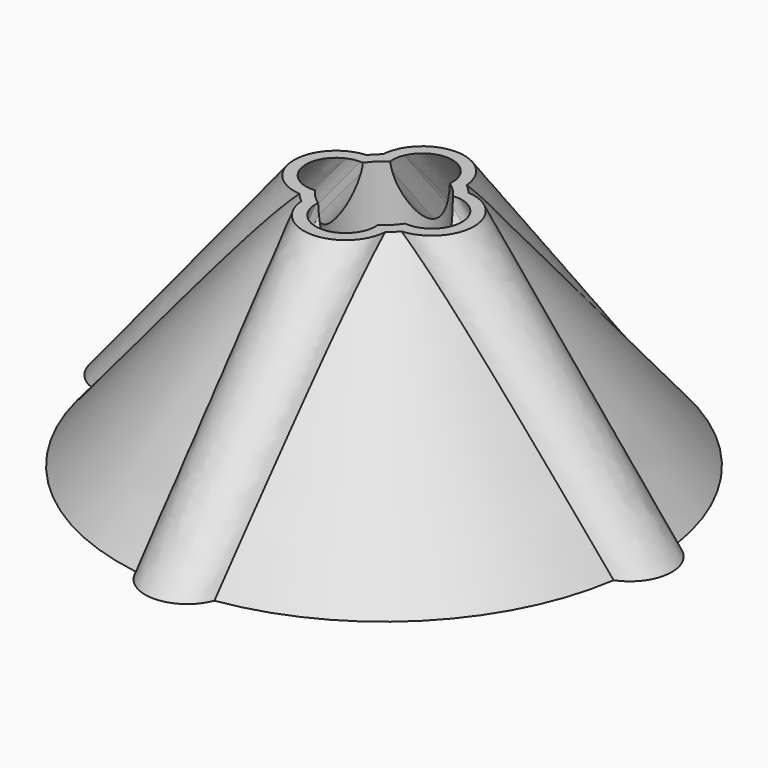
from build123d import *

# Parameters (mm, degrees)
F7_COUNT  = 4
F8_COUNT  = 4
F10_R     = 0.9
F11_DEPTH = 4


with BuildPart() as f1:
    # F0 (on Front) → F1 (revolve)
    with BuildSketch(Plane.XZ):
        Polygon((-0.8, 0), (-0.8, 4), (-1.1, 4), (-4.4, 0), align=None)
    revolve(axis=Axis((0, 0, 2), (0, 0, 1)))

    # F5: sweep along a path in F4
    with BuildLine(Plane(origin=(0, 0, 0), x_dir=(0, -1, 0), z_dir=(-1, 0, 0))) as f5_path:
        Line((-4.4, 0), (-1.1, 4))
    # F2 (on face) → F5 (sweep)
    with BuildSketch(Plane.XY.offset(4)):
        with BuildLine():
            ThreePointArc((0.4582575695, 1), (0.5830784403, 0.9327483757), (0.6982120022, 0.85))
            ThreePointArc((0.6982120022, 0.85), (0, 1.5), (-0.6982120022, 0.85))
            ThreePointArc((-0.6982120022, 0.85), (-0.5830784403, 0.9327483757), (-0.4582575695, 1))
            ThreePointArc((-0.4582575695, 1), (0, 1.3), (0.4582575695, 1))
        make_face()
        with BuildLine():
            ThreePointArc((-0.4582575695, 1), (-0.5830784403, 0.9327483757), (-0.6982120022, 0.85))
            ThreePointArc((-0.6982120022, 0.85), (-0.6873150882, 0.667342661), (-0.6294528874, 0.49375))
            ThreePointArc((-0.6294528874, 0.49375), (-0.5572758185, 0.5739718304), (-0.4749588798, 0.64375))
            ThreePointArc((-0.4749588798, 0.64375), (-0.49945145, 0.823414719), (-0.4582575695, 1))
        make_face()
        with BuildLine():
            ThreePointArc((-0.6294528874, 0.49375), (0, 0.1), (0.6294528874, 0.49375))
            ThreePointArc((0.6294528874, 0.49375), (0.5572758185, 0.5739718304), (0.4749588798, 0.64375))
            ThreePointArc((0.4749588798, 0.64375), (0, 0.3), (-0.4749588798, 0.64375))
            ThreePointArc((-0.4749588798, 0.64375), (-0.5572758185, 0.5739718304), (-0.6294528874, 0.49375))
        make_face()
        with BuildLine():
            ThreePointArc((0.6294528874, 0.49375), (0.6821352583, 0.6428647417), (0.7, 0.8))
            ThreePointArc((0.7, 0.8), (0.6995528577, 0.8250159796), (0.6982120022, 0.85))
            ThreePointArc((0.6982120022, 0.85), (0.5830784403, 0.9327483757), (0.4582575695, 1))
            ThreePointArc((0.4582575695, 1), (0.4894531565, 0.9021548218), (0.5, 0.8))
            ThreePointArc((0.5, 0.8), (0.4937000303, 0.7208780685), (0.4749588798, 0.64375))
            ThreePointArc((0.4749588798, 0.64375), (0.5572758185, 0.5739718304), (0.6294528874, 0.49375))
        make_face()
    sweep(path=f5_path.line)

    # F6: sweep along a path in F4
    with BuildLine(Plane(origin=(0, 0, 0), x_dir=(0, -1, 0), z_dir=(-1, 0, 0))) as f6_path:
        Line((-4.4, 0), (-1.1, 4))
    # F2 (on face) → F6 (sweep, cut)
    with BuildSketch(Plane.XY.offset(4)):
        with BuildLine():
            ThreePointArc((-0.4582575695, 1), (0, 1.1), (0.4582575695, 1))
            ThreePointArc((0.4582575695, 1), (0, 1.3), (-0.4582575695, 1))
        make_face()
        with BuildLine():
            ThreePointArc((-0.4749588798, 0.64375), (0, 0.3), (0.4749588798, 0.64375))
            ThreePointArc((0.4749588798, 0.64375), (0, 0.8), (-0.4749588798, 0.64375))
        make_face()
        with BuildLine():
            ThreePointArc((0.5, 0.8), (0.4894531565, 0.9021548218), (0.4582575695, 1))
            ThreePointArc((0.4582575695, 1), (0, 1.1), (-0.4582575695, 1))
            ThreePointArc((-0.4582575695, 1), (-0.49945145, 0.823414719), (-0.4749588798, 0.64375))
            ThreePointArc((-0.4749588798, 0.64375), (0, 0.8), (0.4749588798, 0.64375))
            ThreePointArc((0.4749588798, 0.64375), (0.4937000303, 0.7208780685), (0.5, 0.8))
        make_face()
    f6 = sweep(path=f6_path.line, mode=Mode.SUBTRACT)

    # F7: F6 ×4 about axis
    f7_axis = Axis((0, 0, 4), (0, 0, -1))
    for i in range(1, F7_COUNT):
        add(f6.rotate(f7_axis, i * 360 / F7_COUNT), mode=Mode.SUBTRACT)


with BuildPart() as f8_1:
    # F8: instance of F1
    add(f1.part.rotate(Axis((0, 0, 0), (0, 0, 1)), 1 * 360 / F8_COUNT))


with BuildPart() as f8_2:
    # F8: instance of F1
    add(f1.part.rotate(Axis((0, 0, 0), (0, 0, 1)), 2 * 360 / F8_COUNT))


with BuildPart() as f8_3:
    # F8: instance of F1
    add(f1.part.rotate(Axis((0, 0, 0), (0, 0, 1)), 3 * 360 / F8_COUNT))


with BuildPart() as f8_2_1:
    add(f8_2.part)

    # F9: union F8_3, F1, F8_1
    add(f8_3.part)
    add(f1.part)
    add(f8_1.part)

    # F10 (on face) → F11 (cut)
    with BuildSketch(Plane(origin=(0, 0, 0), x_dir=(1, 0, 0), z_dir=(0, 0, -1))):
        Circle(F10_R)
    extrude(amount=-F11_DEPTH, mode=Mode.SUBTRACT)


solid = f8_2_1.part
